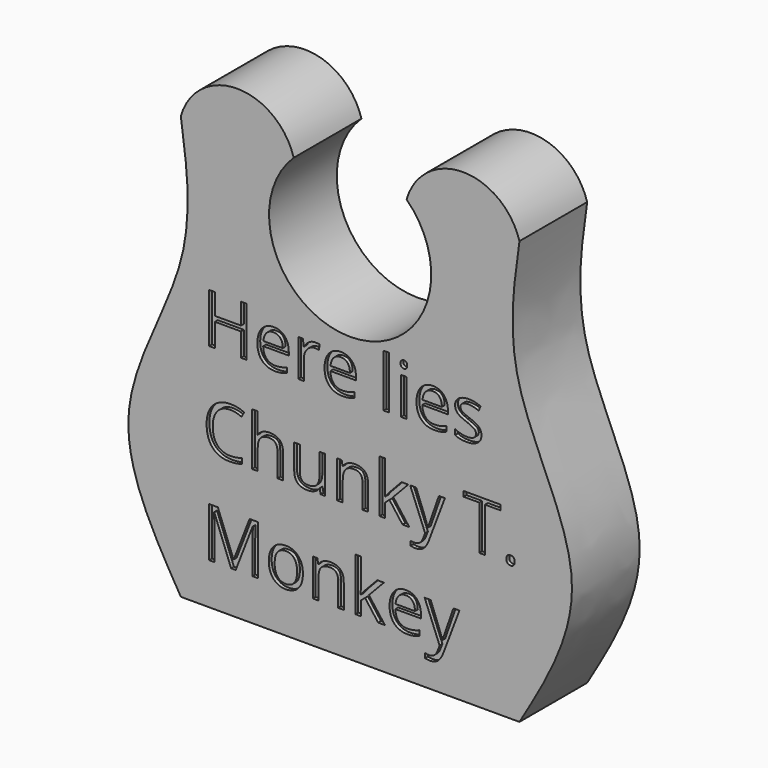
from build123d import *

# Parameters (mm, degrees)
F1_DEPTH     = 152.4
F2_TEXT_SIZE = 124.7636146016
F3_DEPTH     = 6.35


# Not quite as in the source:
# - Text() gives the source's letters only with a copy of the font that has no kerning and outlines rounded to 1/6400 em; it was checked with that copy


with BuildPart() as f1:
    # F0 (on Front) → F1 (new body)
    with BuildSketch(Plane.XZ):
        with BuildLine():
            add(Edge.make_bspline(
                [(-482.8187534992, 762), (-472.1962511564, 687.1427651202), (-449.5900125157, 527.8356206198), (-633.8256428282, 255.7547164043), (-532.6201062407, 84.3466871183), (-482.8187534992, 0)],
                knots=[0, 0, 0, 0, 0.3104514229, 0.6606860348, 1, 1, 1, 1], degree=3))
            Line((-482.8187534992, 0), (126.7812465008, 0))
            add(Edge.make_bspline(
                [(126.7812465008, 762), (116.158744158, 687.1427651202), (93.5525055173, 527.8356206198), (277.7881358298, 255.7547164043), (176.5825992422, 84.3466871183), (126.7812465008, 0)],
                knots=[0, 0, 0, 0, 0.3104514229, 0.6606860348, 1, 1, 1, 1], degree=3))
            ThreePointArc((126.7812465008, 762), (25.1812465008, 838.5503412308), (-76.4187534992, 762))
            ThreePointArc((-76.4187534992, 762), (-178.0187534992, 511.2056971825), (-279.6187534992, 762))
            ThreePointArc((-279.6187534992, 762), (-381.2187534992, 838.5503412308), (-482.8187534992, 762))
        make_face()
    extrude(amount=F1_DEPTH)

    # F2 (on face) → F3 (cut)
    with BuildSketch(Plane.XZ.offset(152.4)):
        with Locations((-444.0531432629, 413.9975607395)):
            Text('Here lies', F2_TEXT_SIZE, font='Open Sans', text_align=(TextAlign.LEFT, TextAlign.BOTTOM))
        with Locations((-444.0531432629, 244.3190448814)):
            Text('Chunky T.', F2_TEXT_SIZE, font='Open Sans', text_align=(TextAlign.LEFT, TextAlign.BOTTOM))
        with Locations((-444.0531432629, 74.6405290233)):
            Text('Monkey', F2_TEXT_SIZE, font='Open Sans', text_align=(TextAlign.LEFT, TextAlign.BOTTOM))
    extrude(amount=-F3_DEPTH, mode=Mode.SUBTRACT)


solid = f1.part
